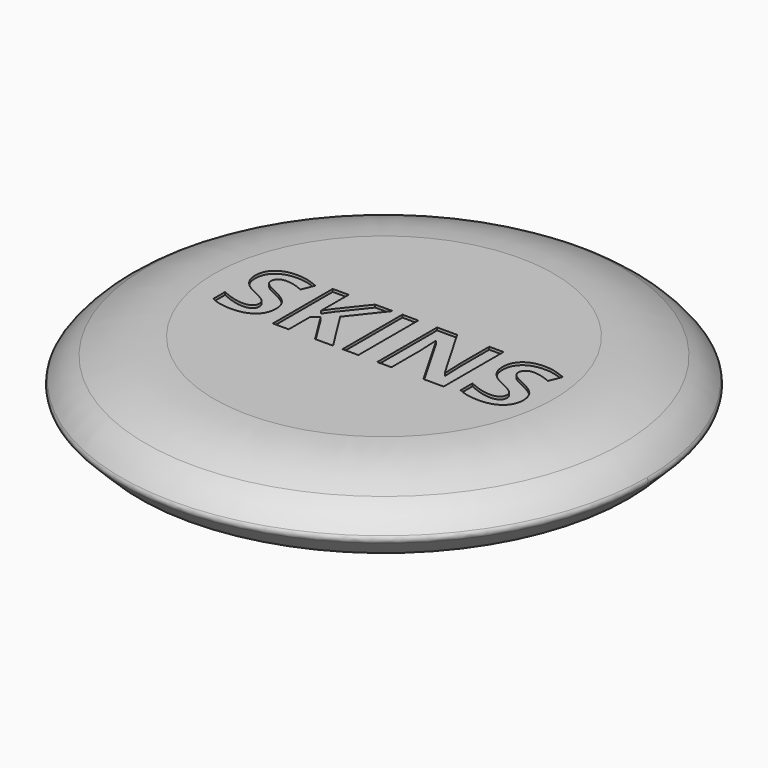
from build123d import *

# Parameters (mm, degrees)
F0_R         = 50
F1_DEPTH     = 12
F2_SIZE      = 4
F5_TEXT_SIZE = 19.7614991482
F6_DEPTH     = 0.5
F9_R         = 1


# Not quite as in the source:
# - Text() gives the source's letters only with a copy of the font that has no kerning and outlines rounded to 1/6400 em; it was checked with that copy


with BuildPart() as f1:
    # F0 (on Top) → F1 (new body)
    with BuildSketch(Plane.XY):
        Circle(F0_R)
    extrude(amount=F1_DEPTH)

    # F2
    f2_edges = [f1.edges().sort_by_distance(p)[0] for p in [
        (-50, 0, 0),
    ]]
    chamfer(f2_edges, length=F2_SIZE)

    # F3 (on Front) → F4 (revolve, cut)
    with BuildSketch(Plane.XZ):
        with BuildLine():
            Line((-50, 12), (-50, 4))
            ThreePointArc((-50, 4), (-47.7685622075, 6.7523700981), (-44.8737123605, 8.7955783943))
            ThreePointArc((-44.8737123605, 8.7955783943), (-38.6245196568, 11.1517242015), (-32, 12))
            Line((-32, 12), (-50, 12))
        make_face()
    revolve(axis=Axis((0, 0, 32.4962362647), (0, 0, 1)), mode=Mode.SUBTRACT)

    # F5 (on face) → F6 (cut)
    with BuildSketch(Plane.XY.offset(12)):
        with Locations((-28, -7.0065842226)):
            Text('SKINS', F5_TEXT_SIZE, font='Open Sans', font_style=FontStyle.BOLD, text_align=(TextAlign.LEFT, TextAlign.BOTTOM))
    extrude(amount=-F6_DEPTH, mode=Mode.SUBTRACT)

    # F7 (on Front) → F8 (revolve, cut)
    with BuildSketch(Plane.XZ):
        with BuildLine():
            Line((-44, 0), (0, 0))
            Line((0, 0), (0, 9))
            ThreePointArc((0, 9), (-22.4564280989, 6.7314262612), (-44, 0))
        make_face()
    revolve(axis=Axis((0, 0, -15.0621237699), (0, 0, 1)), mode=Mode.SUBTRACT)

    # F9
    f9_edges = [f1.edges().sort_by_distance(p)[0] for p in [
        (0, -50, 4),
        (0, 50, 4),
    ]]
    fillet(f9_edges, radius=F9_R)


solid = f1.part
